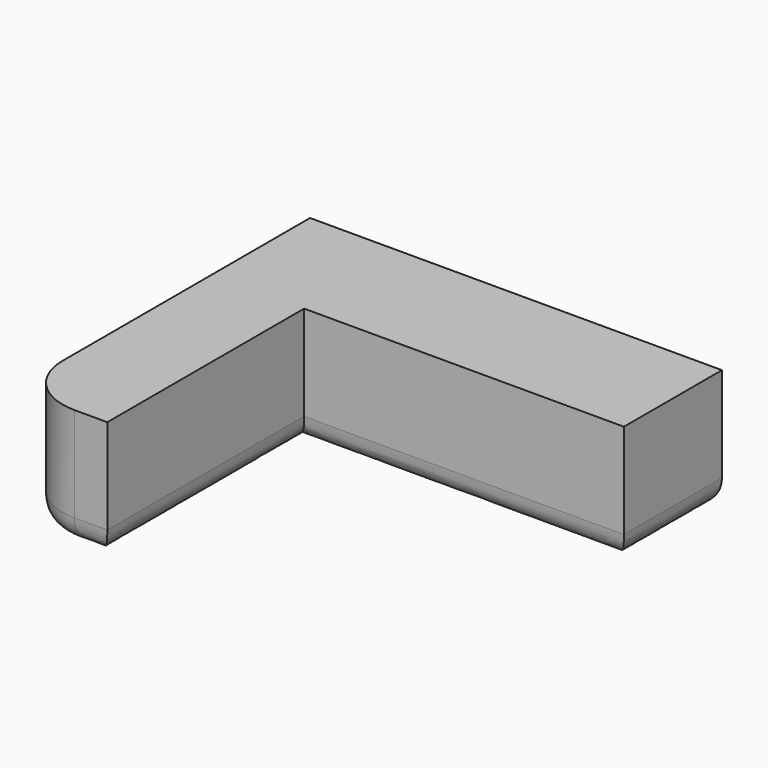
from build123d import *

# Parameters (mm, degrees)
F1_DEPTH     = 25.4
F2_T1_DEPTH  = 78.9172077388
F2_T3_DEPTH  = 19.7233948857
F2_T5_DEPTH  = 65.3813702494
F2_T7_DEPTH  = 81.1736724943
F2_T9_DEPTH  = 51.6358374894
F2_T11_DEPTH = 113.59706738
F2_T14_ANGLE = 90
F2_T19_DEPTH = 93.8736724943
F2_T23_DEPTH = 78.0813702494


# Not quite as in the source:
# - a fillet or chamfer that OpenCascade refuses, or shapes differently, is made with other operations: its cross-section is extruded or revolved along the edge and cut away or added


with BuildPart() as f1:
    # F0 (on Top) → F1 (new body)
    with BuildSketch(Plane.XY):
        with BuildLine():
            Line((-17.2114539891, 42.8890809417), (-36.9348488748, 42.8890809417))
            Line((-36.9348488748, 42.8890809417), (-36.9348488748, 16.6532434523))
            Line((-36.9348488748, 16.6532434523), (-36.9348488748, -23.3281267971))
            ThreePointArc((-36.9348488748, -23.3281267971), (-33.2151049959, -32.3083829181), (-24.2348488748, -36.0281267971))
            Line((-24.2348488748, -36.0281267971), (-17.2114539891, -36.0281267971))
            Line((-17.2114539891, -36.0281267971), (-17.2114539891, 16.6532434523))
            Line((-17.2114539891, 16.6532434523), (51.2622185051, 16.6532434523))
            Line((51.2622185051, 16.6532434523), (51.2622185051, 42.8890809417))
            Line((51.2622185051, 42.8890809417), (-17.2114539891, 42.8890809417))
        make_face()
    extrude(amount=F1_DEPTH)

    # F2: fillet of radius 5.08 on 7 edges, made by hand

    # F2_s2 → F2_t1 (cut)
    with BuildSketch(Plane.XZ.offset(-55.5890809417)):
        with BuildLine():
            add(Edge.make_bspline(
                [(-31.8548488748, 0), (-36.9348488748, 0), (-36.9348488748, 5.08)],
                knots=[0, 0, 0, 1, 1, 1], degree=2, weights=[1, 1, 1]))
            Line((-36.9348488748, 5.08), (-36.9348488748, 0))
            Line((-36.9348488748, 0), (-31.8548488748, 0))
        make_face()
    extrude(amount=F2_T1_DEPTH, mode=Mode.SUBTRACT)

    # F2_s4 → F2_t3 (cut)
    with BuildSketch(Plane.YZ.offset(-24.2348488748)):
        with BuildLine():
            add(Edge.make_bspline(
                [(-36.0281267971, 5.08), (-36.0281267971, 0), (-30.9481267971, 0)],
                knots=[0, 0, 0, 1, 1, 1], degree=2, weights=[1, 1, 1]))
            Line((-30.9481267971, 0), (-36.0281267971, 0))
            Line((-36.0281267971, 0), (-36.0281267971, 5.08))
        make_face()
    extrude(amount=F2_T3_DEPTH, mode=Mode.SUBTRACT)

    # F2_s6 → F2_t5 (cut)
    with BuildSketch(Plane.XZ.offset(-16.6532434523)):
        with BuildLine():
            add(Edge.make_bspline(
                [(-17.2114539891, 5.08), (-17.2114539891, 0), (-22.2914539891, 0)],
                knots=[0, 0, 0, 1, 1, 1], degree=2, weights=[1, 1, 1]))
            Line((-22.2914539891, 0), (-17.2114539891, 0))
            Line((-17.2114539891, 0), (-17.2114539891, 5.08))
        make_face()
    extrude(amount=F2_T5_DEPTH, mode=Mode.SUBTRACT)

    # F2_s8 → F2_t7 (cut)
    with BuildSketch(Plane.YZ.offset(-17.2114539891)):
        with BuildLine():
            add(Edge.make_bspline(
                [(16.6532434523, 5.08), (16.6532434523, 0), (21.7332434523, 0)],
                knots=[0, 0, 0, 1, 1, 1], degree=2, weights=[1, 1, 1]))
            Line((21.7332434523, 0), (16.6532434523, 0))
            Line((16.6532434523, 0), (16.6532434523, 5.08))
        make_face()
    extrude(amount=F2_T7_DEPTH, mode=Mode.SUBTRACT)

    # F2_s10 → F2_t9 (cut)
    with BuildSketch(Plane.XZ.offset(-55.5890809417)):
        with BuildLine():
            add(Edge.make_bspline(
                [(51.2622185051, 5.08), (51.2622185051, 0), (46.1822185051, 0)],
                knots=[0, 0, 0, 1, 1, 1], degree=2, weights=[1, 1, 1]))
            Line((46.1822185051, 0), (51.2622185051, 0))
            Line((51.2622185051, 0), (51.2622185051, 5.08))
        make_face()
    extrude(amount=F2_T9_DEPTH, mode=Mode.SUBTRACT)

    # F2_s12 → F2_t11 (cut)
    with BuildSketch(Plane.YZ.offset(-49.6348488748)):
        with BuildLine():
            add(Edge.make_bspline(
                [(42.8890809417, 5.08), (42.8890809417, 0), (37.8090809417, 0)],
                knots=[0, 0, 0, 1, 1, 1], degree=2, weights=[1, 1, 1]))
            Line((37.8090809417, 0), (42.8890809417, 0))
            Line((42.8890809417, 0), (42.8890809417, 5.08))
        make_face()
    extrude(amount=F2_T11_DEPTH, mode=Mode.SUBTRACT)

    # F2_s13 → F2_t14 (revolve, cut)
    with BuildSketch(Plane.XZ.offset(23.3281267971)):
        with BuildLine():
            add(Edge.make_bspline(
                [(-36.9348488748, 5.08), (-36.9348488748, 0), (-31.8548488748, 0)],
                knots=[0, 0, 0, 1, 1, 1], degree=2, weights=[1, 1, 1]))
            Line((-31.8548488748, 0), (-36.9348488748, 0))
            Line((-36.9348488748, 0), (-36.9348488748, 5.08))
        make_face()
    revolve(axis=Axis((-24.2348488748, -23.3281267971, 0), (0, 0, 1)), revolution_arc=F2_T14_ANGLE, mode=Mode.SUBTRACT)


with BuildPart() as f2_tool17:
    # F2_s18 → F2_t19 (new body)
    with BuildSketch(Plane.YZ.offset(-29.9114539891)):
        with BuildLine():
            add(Edge.make_bspline(
                [(16.6532434523, 5.08), (16.6532434523, 0), (21.7332434523, 0)],
                knots=[0, 0, 0, 1, 1, 1], degree=2, weights=[1, 1, 1]))
            Line((21.7332434523, 0), (16.6532434523, 0))
            Line((16.6532434523, 0), (16.6532434523, 5.08))
        make_face()
    extrude(amount=F2_T19_DEPTH)

    split(bisect_by=Plane.YZ.offset(-17.2114539891), keep=Keep.BOTTOM)


with BuildPart() as f2_tool21:
    # F2_s22 → F2_t23 (new body)
    with BuildSketch(Plane.XZ.offset(48.7281267971)):
        with BuildLine():
            add(Edge.make_bspline(
                [(-17.2114539891, 5.08), (-17.2114539891, 0), (-22.2914539891, 0)],
                knots=[0, 0, 0, 1, 1, 1], degree=2, weights=[1, 1, 1]))
            Line((-22.2914539891, 0), (-17.2114539891, 0))
            Line((-17.2114539891, 0), (-17.2114539891, 5.08))
        make_face()
    extrude(amount=-F2_T23_DEPTH)

    split(bisect_by=Plane.XZ.offset(-16.6532434523), keep=Keep.BOTTOM)


with BuildPart() as f2_tool17_1:
    add(f2_tool17.part)

    # F2_t25: intersect F2_tool21
    add(f2_tool21.part, mode=Mode.INTERSECT)


with BuildPart() as f1_1:
    add(f1.part)

    # F2_t15: cut F2_tool17
    add(f2_tool17_1.part, mode=Mode.SUBTRACT)


solid = f1_1.part
